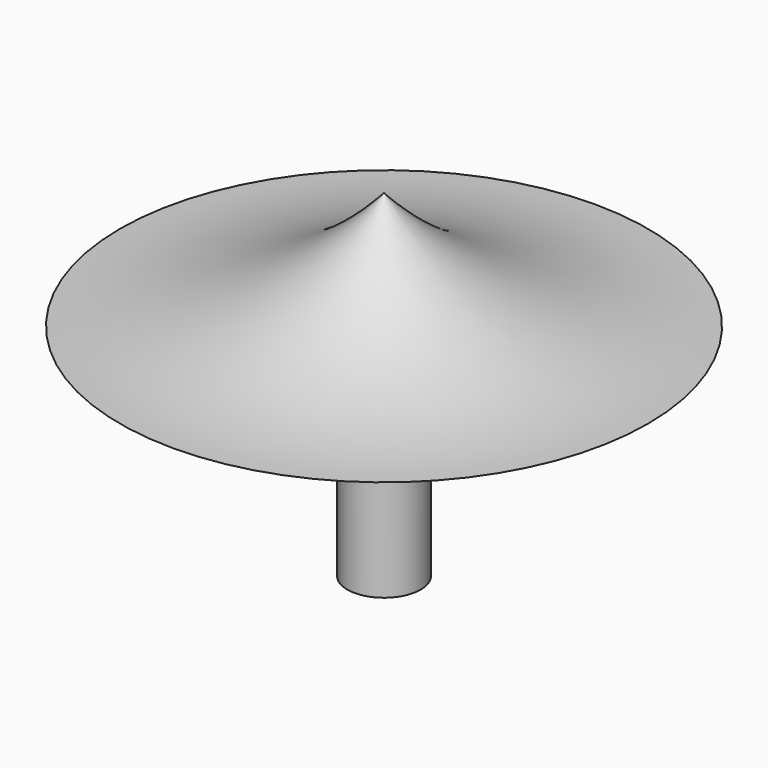
from build123d import *

# Parameters (mm, degrees)
F2_R         = 3.175
F3_DEPTH     = 19.05
F4_TEXT_SIZE = 20.5164931561
F5_DEPTH     = 1.27


# Not quite as in the source:
# - Text() gives the source's letters only with a copy of the font that has no kerning and outlines rounded to 1/6400 em; it was checked with that copy


with BuildPart() as f1:
    # F0 (on Front) → F1 (revolve)
    with BuildSketch(Plane.XZ):
        with BuildLine():
            Line((0, 10.16), (0, 0))
            Line((0, 0), (22.86, 0))
            ThreePointArc((22.86, 0), (10.3519505917, 2.6543888314), (0, 10.16))
        make_face()
    revolve(axis=Axis((0, 0, 5.08), (0, 0, 1)))

    # F2 (on face) → F3 (join)
    with BuildSketch(Plane(origin=(0, 0, 0), x_dir=(1, 0, 0), z_dir=(0, 0, -1))):
        Circle(F2_R)
    extrude(amount=F3_DEPTH)

    # F4 (on face) → F5 (join)
    with BuildSketch(Plane(origin=(0, 0, 0), x_dir=(1, 0, 0), z_dir=(0, 0, -1))):
        with Locations((-11.5279449643, -19.8242826885)):
            Text('S I', F4_TEXT_SIZE, font='Open Sans', font_style=FontStyle.BOLD, text_align=(TextAlign.LEFT, TextAlign.BOTTOM))
    extrude(amount=F5_DEPTH)


solid = f1.part
